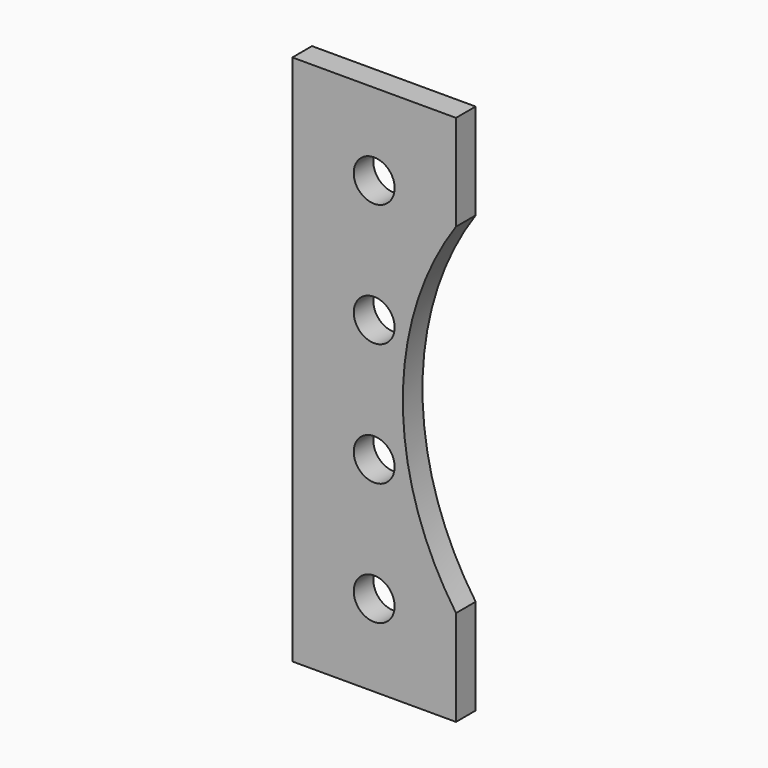
from build123d import *

# Parameters (mm, degrees)
F0_R     = 5
F1_DEPTH = 6


# Not quite as in the source:
# - a feature names something its author has since deleted; it is built from what else it names


with BuildPart() as f1:
    # F0 (on Front) → F1 (new body)
    with BuildSketch(Plane.XZ):
        with BuildLine():
            Line((0, 130), (0, 0))
            Line((0, 0), (40, 0))
            Line((40, 0), (40, 23.4187542274))
            ThreePointArc((40, 23.4187542274), (27, 65), (40, 106.5812457726))
            Line((40, 106.5812457726), (40, 130))
            Line((40, 130), (35, 130))
            Line((35, 130), (0, 130))
        make_face()
        with Locations((20, 20)):
            Circle(F0_R, mode=Mode.SUBTRACT)
        with Locations((20, 50)):
            Circle(F0_R, mode=Mode.SUBTRACT)
        with Locations((20, 80)):
            Circle(F0_R, mode=Mode.SUBTRACT)
        with Locations((20, 110)):
            Circle(F0_R, mode=Mode.SUBTRACT)
    extrude(amount=F1_DEPTH)


solid = f1.part
